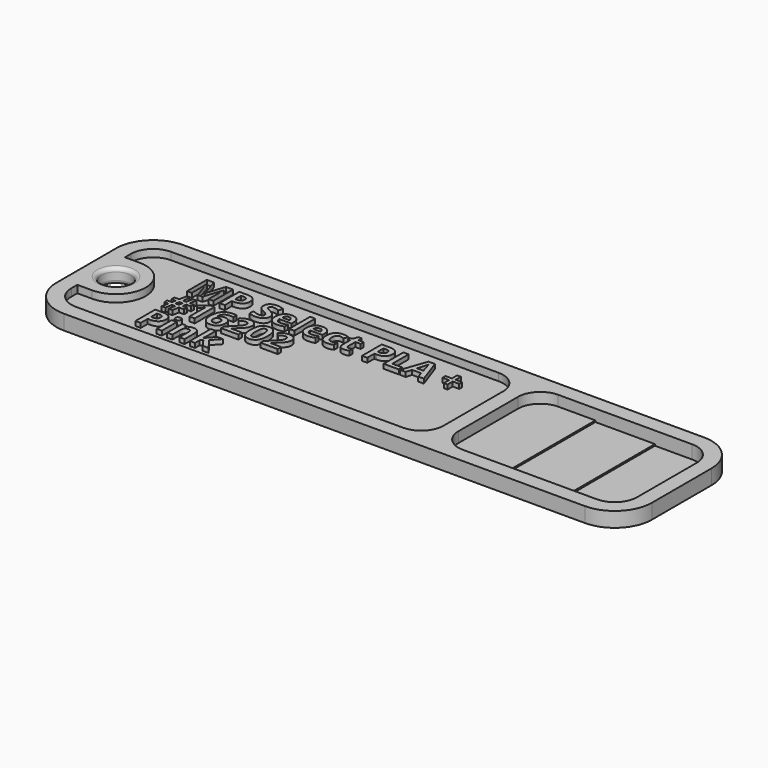
from build123d import *

# Parameters (mm, degrees)
F1_DEPTH      = 2
F3_DEPTH      = 1
F4_R          = 2
F5_DEPTH      = 2.001
F6_R          = 0.5
F7_DEPTH      = 0.4
F9_DEPTH      = 0.2
F11_DEPTH     = 0.2
F12_TEXT_SIZE = 4.6296296296
F13_DEPTH     = 0.6


# Not quite as in the source:
# - Text() gives the source's letters only with a copy of the font that has no kerning and outlines rounded to 1/6400 em; it was checked with that copy


with BuildPart() as f1:
    # F0 (on Top) → F1 (new body)
    with BuildSketch(Plane.XY):
        with BuildLine():
            ThreePointArc((40, 5), (38.5355339059, 8.5355339059), (35, 10))
            Line((35, 10), (-35, 10))
            ThreePointArc((-35, 10), (-38.5355339059, 8.5355339059), (-40, 5))
            Line((-40, 5), (-40, -5))
            ThreePointArc((-40, -5), (-38.5355339059, -8.5355339059), (-35, -10))
            Line((-35, -10), (35, -10))
            ThreePointArc((35, -10), (38.5355339059, -8.5355339059), (40, -5))
            Line((40, -5), (40, 5))
        make_face()
    extrude(amount=F1_DEPTH)

    # F2 (on face) → F3 (cut)
    with BuildSketch(Plane.XY.offset(2)):
        with BuildLine():
            ThreePointArc((35, -8), (37.1213203436, -7.1213203436), (38, -5))
            Line((38, -5), (38, 5))
            ThreePointArc((38, 5), (37.1213203436, 7.1213203436), (35, 8))
            Line((35, 8), (17, 8))
            ThreePointArc((17, 8), (14.8786796564, 7.1213203436), (14, 5))
            Line((14, 5), (14, -5))
            ThreePointArc((14, -5), (14.8786796564, -7.1213203436), (17, -8))
            Line((17, -8), (35, -8))
        make_face()
        with BuildLine():
            ThreePointArc((-38, -5), (-37.1213203436, -7.1213203436), (-35, -8))
            Line((-35, -8), (9, -8))
            ThreePointArc((9, -8), (11.1213203436, -7.1213203436), (12, -5))
            Line((12, -5), (12, 5))
            ThreePointArc((12, 5), (11.1213203436, 7.1213203436), (9, 8))
            Line((9, 8), (-35, 8))
            ThreePointArc((-35, 8), (-37.1213203436, 7.1213203436), (-38, 5))
            Line((-38, 5), (-38, 4))
            Line((-38, 4), (-36, 4))
            ThreePointArc((-36, 4), (-32, 0), (-36, -4))
            Line((-36, -4), (-38, -4))
            Line((-38, -4), (-38, -5))
        make_face()
    extrude(amount=-F3_DEPTH, mode=Mode.SUBTRACT)

    # F4 (on face) → F5 (cut, through all)
    with BuildSketch(Plane.XY.offset(2)):
        with Locations((-36, 0)):
            Circle(F4_R)
    extrude(amount=-F5_DEPTH, mode=Mode.SUBTRACT)

    # F6
    f6_edges = [f1.edges().sort_by_distance(p)[0] for p in [
        (-38, 0, 2),
        (-38, 0, 0),
    ]]
    fillet(f6_edges, radius=F6_R)

    # F7 (cut): a face of the model
    f7_faces = [f1.faces().sort_by_distance(p)[0] for p in [
        (26, 0, 1),
    ]]
    extrude(f7_faces, amount=-F7_DEPTH, mode=Mode.SUBTRACT)

    # F8 (on face) → F9 (cut)
    with BuildSketch(Plane.XY.offset(0.6)):
        with BuildLine():
            Line((22, -8), (35, -8))
            ThreePointArc((35, -8), (37.1213203436, -7.1213203436), (38, -5))
            Line((38, -5), (38, 5))
            ThreePointArc((38, 5), (37.1213203436, 7.1213203436), (35, 8))
            Line((35, 8), (22, 8))
            Line((22, 8), (22, -8))
        make_face()
    extrude(amount=-F9_DEPTH, mode=Mode.SUBTRACT)

    # F10 (on face) → F11 (cut)
    with BuildSketch(Plane.XY.offset(0.4)):
        with BuildLine():
            ThreePointArc((38, 5), (37.1213203436, 7.1213203436), (35, 8))
            Line((35, 8), (30, 8))
            Line((30, 8), (30, -8))
            Line((30, -8), (35, -8))
            ThreePointArc((35, -8), (37.1213203436, -7.1213203436), (38, -5))
            Line((38, -5), (38, 5))
        make_face()
    extrude(amount=-F11_DEPTH, mode=Mode.SUBTRACT)

    # F12 (on face) → F13 (join)
    with BuildSketch(Plane.XY.offset(1)):
        with Locations((-29, 2.6666666667)):
            Text('MP Select PLA +', F12_TEXT_SIZE, font='Open Sans', font_style=FontStyle.BOLD, text_align=(TextAlign.LEFT, TextAlign.BOTTOM))
        with Locations((-29, -1.6666666667)):
            Text('#16202', F12_TEXT_SIZE, font='Open Sans', font_style=FontStyle.BOLD, text_align=(TextAlign.LEFT, TextAlign.BOTTOM))
        with Locations((-29, -6)):
            Text('Pink', F12_TEXT_SIZE, font='Open Sans', font_style=FontStyle.BOLD, text_align=(TextAlign.LEFT, TextAlign.BOTTOM))
    extrude(amount=F13_DEPTH)


solid = f1.part
